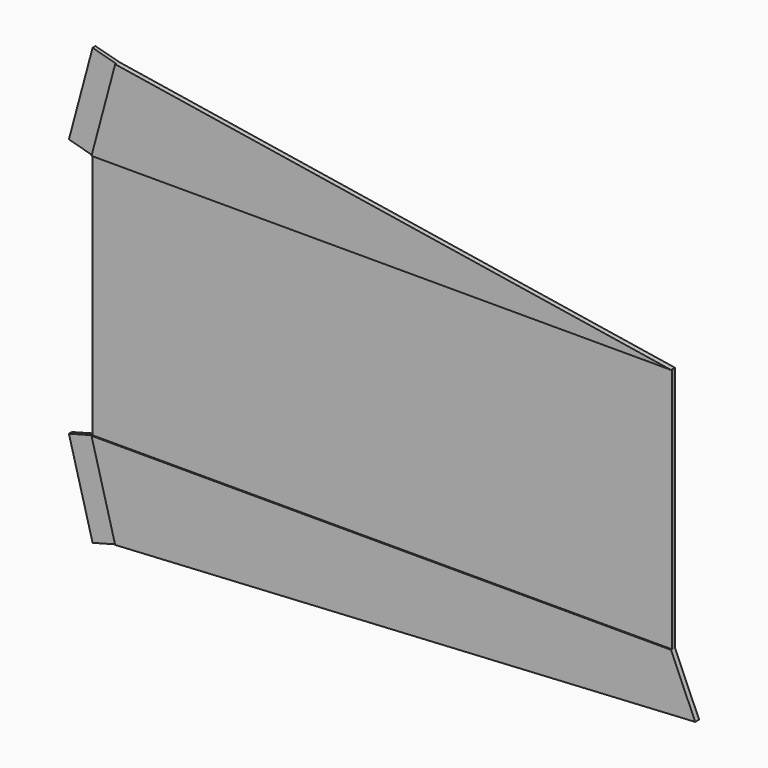
from build123d import *

# Parameters (mm, degrees)
F1_DEPTH = 4
F0_W     = 475
F0_H     = 202
F2_DEPTH = 3


# Not quite as in the source:
# - a feature names something its author has since deleted; it is built from what else it names


with BuildPart() as f1:
    # F0 (on Front) → F1 (new body)
    with BuildSketch(Plane.XZ):
        Polygon((-218.0885716173, 173.4444369717), (-237.5, 101), (237.5, 101), align=None)
    extrude(amount=F1_DEPTH)


with BuildPart() as f1b:
    # F0 (on Front) → F1, piece 2 (new body)
    with BuildSketch(Plane.XZ):
        Polygon((237.5, -101), (-237.5, -101), (-218.0885716173, -173.4444369717), (257.3408484459, -146.5434581041), align=None)
    extrude(amount=F1_DEPTH)


with BuildPart() as f2:
    # F0 (on Front) → F2 (new body)
    with BuildSketch(Plane.XZ):
        Rectangle(F0_W, F0_H)
    extrude(amount=F2_DEPTH)


with BuildPart() as f2b:
    # F0 (on Front) → F2, piece 2 (new body)
    with BuildSketch(Plane.XZ):
        Polygon((-256.8185165258, 106.1763809021), (-237.5, 101), (-218.0885716173, 173.4444369717), (-237.4070881431, 178.6208178737), align=None)
    extrude(amount=F2_DEPTH)


with BuildPart() as f2c:
    # F0 (on Front) → F2, piece 3 (new body)
    with BuildSketch(Plane.XZ):
        Polygon((-218.0885716173, -173.4444369717), (-237.5, -101), (-256.8185165258, -106.1763809021), (-237.4070881431, -178.6208178737), align=None)
    extrude(amount=F2_DEPTH)


solid = Compound([f1.part, f1b.part, f2.part, f2b.part, f2c.part])
